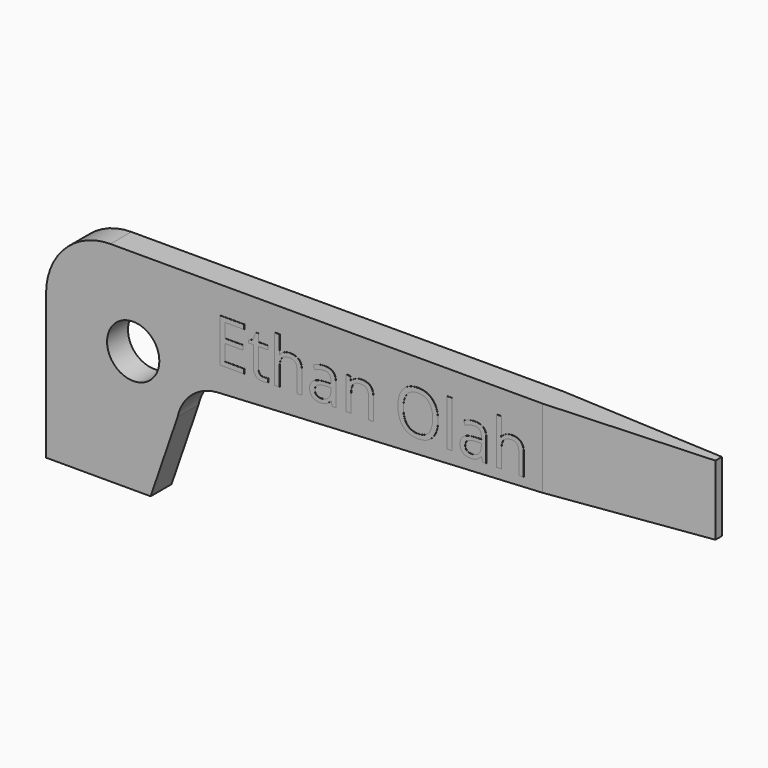
from build123d import *

# Parameters (mm, degrees)
F1_DEPTH     = 2.38125
F2_R         = 2.38125
F3_DEPTH     = 2.38225
F5_DEPTH     = 19.051
F6_TEXT_SIZE = 5.5659264843
F7_DEPTH     = 0.0254


# Not quite as in the source:
# - Text() gives the source's letters only with a copy of the font that has no kerning and outlines rounded to 1/6400 em; it was checked with that copy


with BuildPart() as f1:
    # F0 (on Front) → F1 (new body)
    with BuildSketch(Plane.XZ):
        with BuildLine():
            Line((60.325, 19.05), (5.8674, 19.05))
            ThreePointArc((5.8674, 19.05), (1.7185216721, 17.3314783279), (0, 13.1826))
            Line((0, 13.1826), (0, 0))
            Line((0, 0), (9.525, 0))
            Line((9.525, 0), (11.9859291673, 7.1725254212))
            ThreePointArc((11.9859291673, 7.1725254212), (13.2905001009, 9.3702285148), (15.6634210502, 10.3194652484))
            Line((15.6634210502, 10.3194652484), (60.325, 12.7))
            Line((60.325, 12.7), (60.325, 19.05))
        make_face()
    extrude(amount=F1_DEPTH)

    # F2 (on face) → F3 (cut, through all)
    with BuildSketch(Plane.XZ.offset(2.38125)):
        with Locations((7.9375, 11.1125)):
            Circle(F2_R)
    extrude(amount=-F3_DEPTH, mode=Mode.SUBTRACT)

    # F4 (on face) → F5 (cut, through all)
    with BuildSketch(Plane.XY.offset(19.05)):
        Polygon((60.325, -2.38125), (60.325, -1.5618951613), (45.24375, -2.38125), align=None)
        Polygon((60.325, 0), (45.24375, 0), (60.325, -0.8193548387), align=None)
    extrude(amount=-F5_DEPTH, mode=Mode.SUBTRACT)

    # F6 (on face) → F7 (join)
    with BuildSketch(Plane.XZ.offset(2.38125)):
        with Locations((15.3002804145, 12.6015478745)):
            Text('Ethan Olah', F6_TEXT_SIZE, font='Open Sans', text_align=(TextAlign.LEFT, TextAlign.BOTTOM))
    extrude(amount=F7_DEPTH)


solid = f1.part
